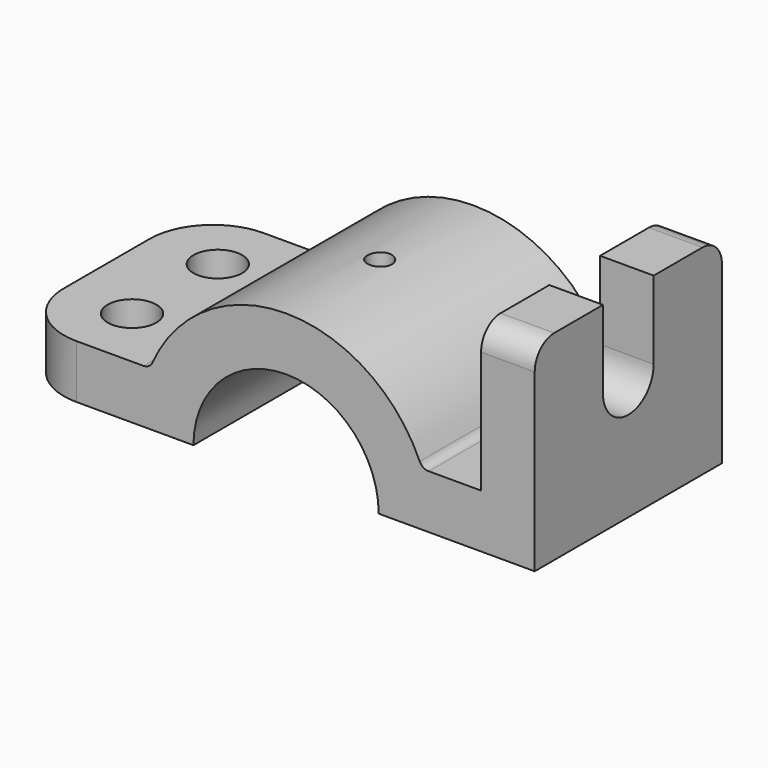
from build123d import *

# Parameters (mm, degrees)
F0_W     = 11
F0_H     = 30
F1_DEPTH = 24
F3_DEPTH = 11
F4_R     = 5
F4_R_2   = 2.5
F5_DEPTH = 41.001
F6_R     = 13
F7_R     = 5
F8_R     = 2


with BuildPart() as f1:
    # F0 (on Front) → F1 (new body, symmetric)
    with BuildSketch(Plane.XZ):
        with BuildLine():
            ThreePointArc((15.4919333848, 11), (18.1017503893, 5.7729223833), (19, 0))
            Line((19, 0), (30, 0))
            ThreePointArc((30, 0), (29.4730143031, 5.5983415304), (27.9105714739, 11))
            Line((27.9105714739, 11), (15.4919333848, 11))
        make_face()
        with BuildLine():
            ThreePointArc((-15.4919333848, 11), (0, 19), (15.4919333848, 11))
            Line((15.4919333848, 11), (27.9105714739, 11))
            ThreePointArc((27.9105714739, 11), (0, 30), (-27.9105714739, 11))
            Line((-27.9105714739, 11), (-15.4919333848, 11))
        make_face()
        with BuildLine():
            Line((-30, 0), (-19, 0))
            ThreePointArc((-19, 0), (-18.1017503893, 5.7729223833), (-15.4919333848, 11))
            Line((-15.4919333848, 11), (-27.9105714739, 11))
            ThreePointArc((-27.9105714739, 11), (-29.4730143031, 5.5983415304), (-30, 0))
        make_face()
        with BuildLine():
            ThreePointArc((27.9105714739, 11), (29.4730143031, 5.5983415304), (30, 0))
            Line((30, 0), (51, 0))
            Line((51, 0), (51, 11))
            Line((51, 11), (40, 11))
            Line((40, 11), (27.9105714739, 11))
        make_face()
        with BuildLine():
            Line((-56, 0), (-30, 0))
            ThreePointArc((-30, 0), (-29.4730143031, 5.5983415304), (-27.9105714739, 11))
            Line((-27.9105714739, 11), (-56, 11))
            Line((-56, 11), (-56, 0))
        make_face()
        with Locations((45.5, 26)):
            Rectangle(F0_W, F0_H)
    extrude(amount=F1_DEPTH, both=True)

    # F2 (on face) → F3 (cut, through all)
    with BuildSketch(Plane.YZ.offset(51)):
        with BuildLine():
            ThreePointArc((-6.5, 25), (0, 31.5), (6.5, 25))
            Line((6.5, 25), (6.5, 41))
            Line((6.5, 41), (-6.5, 41))
            Line((-6.5, 41), (-6.5, 25))
        make_face()
        with BuildLine():
            ThreePointArc((-6.5, 25), (0, 18.5), (6.5, 25))
            ThreePointArc((6.5, 25), (0, 31.5), (-6.5, 25))
        make_face()
    extrude(amount=-F3_DEPTH, mode=Mode.SUBTRACT)

    # F4 (on Top) → F5 (cut, through all)
    with BuildSketch(Plane.XY):
        with Locations((-42, 11)):
            Circle(F4_R)
        with Locations((-42, -11)):
            Circle(F4_R)
        Circle(F4_R_2)
    extrude(amount=F5_DEPTH, mode=Mode.SUBTRACT)

    # F6
    f6_edges = [f1.edges().sort_by_distance(p)[0] for p in [
        (-56, -24, 5.5),
        (-56, 24, 5.5),
    ]]
    fillet(f6_edges, radius=F6_R)

    # F7
    f7_edges = [f1.edges().sort_by_distance(p)[0] for p in [
        (45.5, 24, 41),
        (45.5, -24, 41),
    ]]
    fillet(f7_edges, radius=F7_R)

    # F8
    f8_edges = [f1.edges().sort_by_distance(p)[0] for p in [
        (-27.910571, 0, 11),
        (27.910571, 0, 11),
    ]]
    fillet(f8_edges, radius=F8_R)


solid = f1.part
